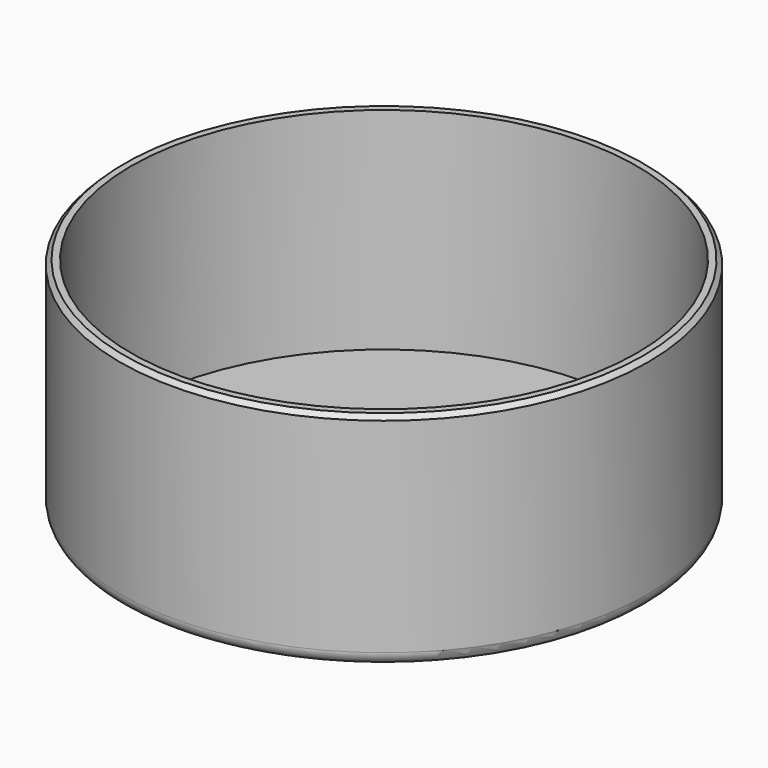
from build123d import *

# Parameters (mm, degrees)
F0_R           = 59.5
F1_DEPTH       = 50
F2_T           = -2.5
F3_R           = 3
F4_R           = 44.5
F4_TEXT_SIZE   = 29.2763178651
F4_TEXT_SIZE_2 = 28.2475105719
F4_TEXT_SIZE_3 = 27.6315789152
F5_DEPTH       = 1
F6_SIZE        = 1


# Not quite as in the source:
# - Text() gives the source's letters only with a copy of the font that has no kerning and outlines rounded to 1/6400 em; it was checked with that copy


with BuildPart() as f1:
    # F0 (on Top) → F1 (new body)
    with BuildSketch(Plane.XY):
        Circle(F0_R)
    extrude(amount=F1_DEPTH)

    # F2
    f2_openings = [f1.faces().sort_by_distance(p)[0] for p in [
        (0, 0, 50),
    ]]
    offset(amount=F2_T, openings=f2_openings)

    # F3
    f3_edges = [f1.edges().sort_by_distance(p)[0] for p in [
        (-59.5, 0, 0),
    ]]
    fillet(f3_edges, radius=F3_R)

    # F4 (on face) → F5 (cut)
    with BuildSketch(Plane(origin=(0, 0, 0), x_dir=(1, 0, 0), z_dir=(0, 0, -1))):
        Circle(F4_R)
        with BuildLine():
            ThreePointArc((37.2958897161, 20.3780914289), (41.1784246477, 10.5160517084), (42.5, 0))
            ThreePointArc((42.5, 0), (30.4035359786, -29.6963802508), (1, -42.4882336653))
            ThreePointArc((1, -42.4882336653), (0, -42.5), (-1, -42.4882336653))
            ThreePointArc((-1, -42.4882336653), (-36.8060796608, -21.25), (-37.2958897161, 20.3780914289))
            ThreePointArc((-37.2958897161, 20.3780914289), (-36.8060796608, 21.25), (-36.2958897161, 22.1101422365))
            ThreePointArc((-36.2958897161, 22.1101422365), (0, 42.5), (36.2958897161, 22.1101422365))
            ThreePointArc((36.2958897161, 22.1101422365), (36.8060796608, 21.25), (37.2958897161, 20.3780914289))
        make_face(mode=Mode.SUBTRACT)
        with BuildLine():
            Line((1, -0.5773502692), (37.2958897161, 20.3780914289))
            ThreePointArc((37.2958897161, 20.3780914289), (36.8060796608, 21.25), (36.2958897161, 22.1101422365))
            Line((36.2958897161, 22.1101422365), (0, 1.1547005384))
            Line((0, 1.1547005384), (-36.2958897161, 22.1101422365))
            ThreePointArc((-36.2958897161, 22.1101422365), (-36.8060796608, 21.25), (-37.2958897161, 20.3780914289))
            Line((-37.2958897161, 20.3780914289), (-1, -0.5773502692))
            Line((-1, -0.5773502692), (-1, -42.4882336653))
            ThreePointArc((-1, -42.4882336653), (0, -42.5), (1, -42.4882336653))
            Line((1, -42.4882336653), (1, -0.5773502692))
        make_face()
        with Locations((-30.4032191634, -22.3971046507)):
            Text('P', F4_TEXT_SIZE, font='Open Sans', text_align=(TextAlign.LEFT, TextAlign.BOTTOM))
        with Locations((-12.2876670988, 13.2635878399)):
            Text('M', F4_TEXT_SIZE_2, font='Open Sans', text_align=(TextAlign.LEFT, TextAlign.BOTTOM))
        with Locations((10.0967809558, -21.2128926069)):
            Text('O', F4_TEXT_SIZE_3, font='Open Sans', text_align=(TextAlign.LEFT, TextAlign.BOTTOM))
    extrude(amount=-F5_DEPTH, mode=Mode.SUBTRACT)

    # F6
    f6_edges = [f1.edges().sort_by_distance(p)[0] for p in [
        (-59.5, 0, 50),
    ]]
    chamfer(f6_edges, length=F6_SIZE)


solid = f1.part
